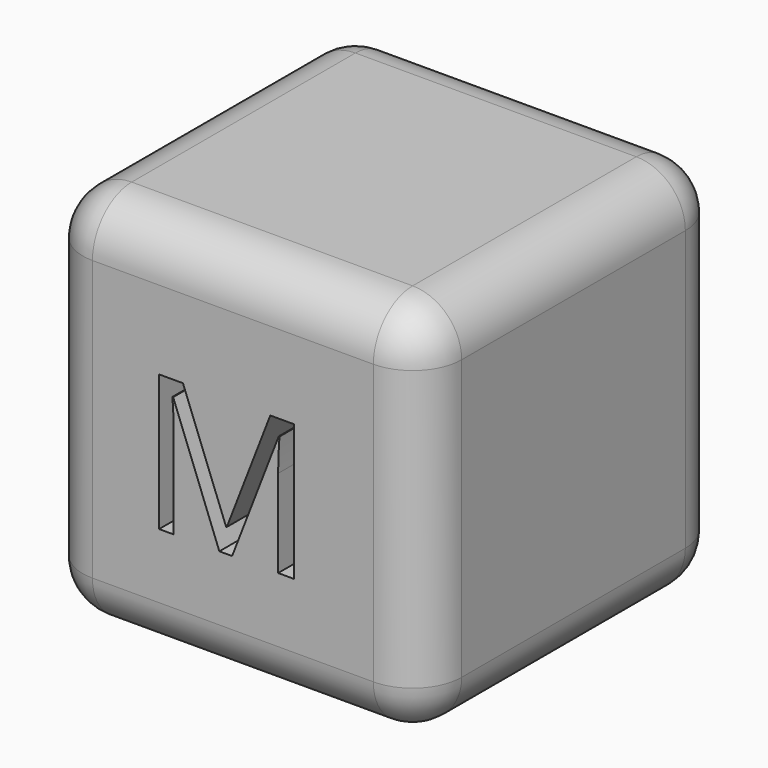
from build123d import *

# Parameters (mm, degrees)
F0_W         = 98.1123447418
F0_H         = 97.7614223957
F1_DEPTH     = 97.7646
F2_R         = 12.7
F3_R         = 12.7
F4_TEXT_SIZE = 100.5063888889
F5_DEPTH     = 6.35
F6_TEXT_SIZE = 49.3768188688
F7_DEPTH     = 12.7


# Not quite as in the source:
# - Text() gives the source's letters only with a copy of the font that has no kerning and outlines rounded to 1/6400 em; it was checked with that copy


with BuildPart() as f1:
    # F0 (on Top) → F1 (new body)
    with BuildSketch(Plane.XY):
        Rectangle(F0_W, F0_H)
    extrude(amount=F1_DEPTH)

    # F2
    f2_edges = [f1.edges().sort_by_distance(p)[0] for p in [
        (0, 48.880711, 97.7646),
    ]]
    fillet(f2_edges, radius=F2_R)

    # F3
    f3_edges = [f1.edges().sort_by_distance(p)[0] for p in [
        (49.056172, -6.35, 97.7646),
        (49.056172, -48.880711, 48.8823),
        (49.056172, 0, 0),
        (49.056172, 48.880711, 42.5323),
        (0, -48.880711, 97.7646),
        (0, -48.880711, 0),
        (0, 48.880711, 0),
        (-49.056172, 0, 0),
        (-49.056172, 48.880711, 42.5323),
        (-49.056172, -48.880711, 48.8823),
        (-49.056172, -6.35, 97.7646),
    ]]
    fillet(f3_edges, radius=F3_R)

    # F4 (on face) → F5 (cut)
    with BuildSketch(Plane.XZ.offset(48.8807111979)):
        with Locations((-36.3561723709, 12.7)):
            Text('M', F4_TEXT_SIZE, font='Open Sans', text_align=(TextAlign.LEFT, TextAlign.BOTTOM))
        Polygon((-36.3561723709, 12.7), (-26.4939829612, 12.7), (-26.4939829612, 84.4521391927), (-13.9306843501, 84.4521391927), (8.7931820128, 25.2632986111), (9.1857850944, 25.2632986111), (32.0981009364, 84.4521391927), (36.3561723709, 84.4521391927), (36.3561723709, 85.0646), (-36.3561723709, 85.0646), align=None)
    extrude(amount=F5_DEPTH, mode=Mode.SUBTRACT)

    # F6 (on face) → F7 (cut)
    with BuildSketch(Plane.XZ.offset(48.8807111979)):
        with Locations((-23.9583402872, 29.4719785452)):
            Text('M', F6_TEXT_SIZE, font='Open Sans', text_align=(TextAlign.LEFT, TextAlign.BOTTOM))
    extrude(amount=-F7_DEPTH, mode=Mode.SUBTRACT)


solid = f1.part
